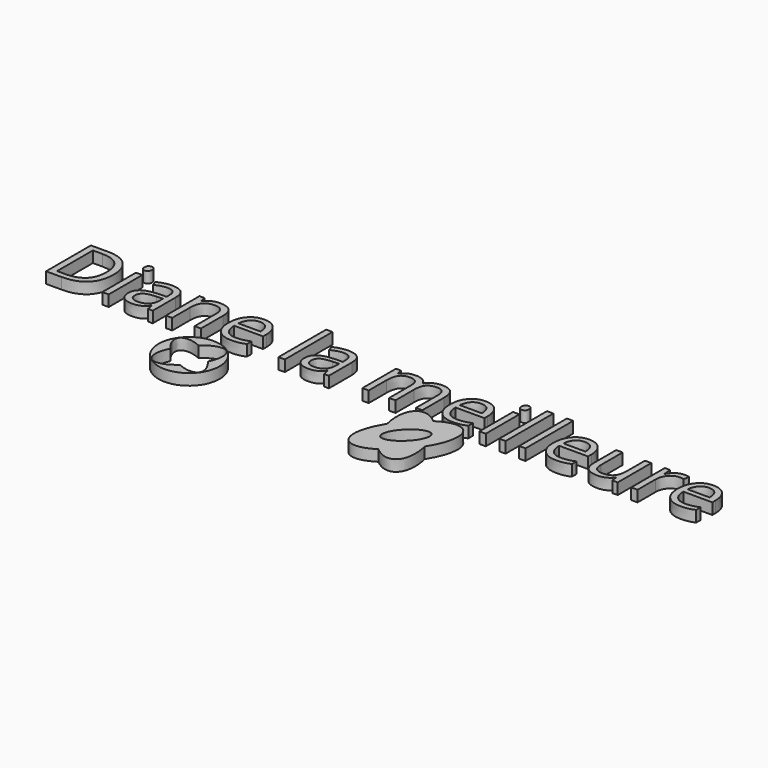
from build123d import *

# Parameters (mm, degrees)
F0_R         = 8.3466025543
F0_TEXT_SIZE = 21.4475266855
F1_DEPTH     = 3.048


# Not quite as in the source:
# - Text() gives the source's letters only with a copy of the font that has no kerning and outlines rounded to 1/6400 em; it was checked with that copy


with BuildPart() as f1:
    # F0 (on Top) → F1 (new body)
    with BuildSketch(Plane.XY):
        with Locations((-38.1957553327, 6.9755995646)):
            Circle(F0_R)
        with BuildLine():
            add(Edge.make_bspline(
                [(-31.5405130386, 2.1061094012), (-30.3175795801, 3.7775202066), (-33.1948879087, 7.1133897692)],
                knots=[0, 0, 0, 1.0706610389, 1.0706610389, 1.0706610389], degree=2, weights=[1, 0.8601000699, 1]))
            add(Edge.make_bspline(
                [(-36.9379521535, 2.2214118859), (-32.788905333, 0.3999034292), (-31.5405130386, 2.1061094012)],
                knots=[5.1943551748, 5.1943551748, 5.1943551748, 6.2831853072, 6.2831853072, 6.2831853072], degree=2, weights=[1, 0.8554303847, 1]))
            add(Edge.make_bspline(
                [(-43.1966227568, 6.83780936), (-51.5075734358, -10.4222102206), (-36.9379521535, 2.2214118859)],
                knots=[1.9673037066, 1.9673037066, 1.9673037066, 4.3401983934, 4.3401983934, 4.3401983934], degree=2, weights=[1, 0.3749556961, 1]))
            add(Edge.make_bspline(
                [(-39.4535585119, 11.7297872433), (-52.2689135199, 17.3559656241), (-43.1966227568, 6.83780936)],
                knots=[2.0527625212, 2.0527625212, 2.0527625212, 4.2122536925, 4.2122536925, 4.2122536925], degree=2, weights=[1, 0.4715527317, 1]))
            add(Edge.make_bspline(
                [(-33.163741231, 13.4682534263), (-35.4280423519, 15.223159111), (-39.4535585119, 11.7297872433)],
                knots=[0, 0, 0, 1.1986057398, 1.1986057398, 1.1986057398], degree=2, weights=[1, 0.8257290436, 1]))
            add(Edge.make_bspline(
                [(-33.1948879087, 7.1133897692), (-30.9580635514, 11.7587827808), (-33.163741231, 13.4682534263)],
                knots=[5.1088963602, 5.1088963602, 5.1088963602, 6.2831853072, 6.2831853072, 6.2831853072], degree=2, weights=[1, 0.8325259928, 1]))
        make_face(mode=Mode.SUBTRACT)
        with BuildLine():
            add(Edge.make_bspline(
                [(21.5702417091, 15.7017175195), (18.5557697987, 18.365754121), (16.3447521627, 17.363846302)],
                knots=[5.4576286446, 5.4576286446, 5.4576286446, 6.2831853072, 6.2831853072, 6.2831853072], degree=2, weights=[1, 0.9160098158, 1]))
            add(Edge.make_bspline(
                [(16.3447521627, 17.363846302), (12.8807705497, 15.7941662569), (14.6476925008, 8.579263006)],
                knots=[0, 0, 0, 1.2026913641, 1.2026913641, 1.2026913641], degree=2, weights=[1, 0.8245750386, 1]))
            add(Edge.make_bspline(
                [(21.5702417091, 15.7017175195), (17.5353416488, 13.1471373461), (14.6476925008, 8.579263006)],
                knots=[0.9615181834, 0.9615181834, 0.9615181834, 1.7930053986, 1.7930053986, 1.7930053986], degree=2, weights=[1, 0.9148162524, 1]))
        make_face()
        with BuildLine():
            add(Edge.make_bspline(
                [(21.5702417091, 15.7017175195), (17.5353416488, 13.1471373461), (14.6476925008, 8.579263006)],
                knots=[0.9615181834, 0.9615181834, 0.9615181834, 1.7930053986, 1.7930053986, 1.7930053986], degree=2, weights=[1, 0.9148162524, 1]))
            add(Edge.make_bspline(
                [(14.6476925008, 8.579263006), (16.2503369357, 2.0351570048), (20.5339913472, -1.7505183903)],
                knots=[1.2026913641, 1.2026913641, 1.2026913641, 2.316035991, 2.316035991, 2.316035991], degree=2, weights=[1, 0.8490180379, 1]))
            add(Edge.make_bspline(
                [(20.5339913472, -1.7505183903), (24.5688914075, 0.8040617832), (27.4565405555, 5.3719361233)],
                knots=[4.103110837, 4.103110837, 4.103110837, 4.9345980522, 4.9345980522, 4.9345980522], degree=2, weights=[1, 0.9148162524, 1]))
            add(Edge.make_bspline(
                [(27.4565405555, 5.3719361233), (25.8538961206, 11.9160421244), (21.5702417091, 15.7017175195)],
                knots=[4.3442840177, 4.3442840177, 4.3442840177, 5.4576286446, 5.4576286446, 5.4576286446], degree=2, weights=[1, 0.8490180379, 1]))
        make_face()
        with BuildLine():
            add(Edge.make_bspline(
                [(17.1563643962, 3.0800073873), (20.3425774952, -0.1063365389), (24.5930991436, 7.3302236901), (28.843620792, 14.7667839192), (21.4068860446, 10.5165676164), (13.9701512972, 6.2663513136), (17.1563643962, 3.0800073873)],
                knots=[0, 0, 0, 2.0943951024, 2.0943951024, 4.1887902048, 4.1887902048, 6.2831853072, 6.2831853072, 6.2831853072], degree=2, weights=[1, 0.5, 1, 0.5, 1, 0.5, 1]))
        make_face(mode=Mode.SUBTRACT)
        with BuildLine():
            add(Edge.make_bspline(
                [(14.6476925008, 8.579263006), (16.2503369357, 2.0351570048), (20.5339913472, -1.7505183903)],
                knots=[1.2026913641, 1.2026913641, 1.2026913641, 2.316035991, 2.316035991, 2.316035991], degree=2, weights=[1, 0.8490180379, 1]))
            add(Edge.make_bspline(
                [(14.6476925008, 8.579263006), (-0.168217137, -14.8575224175), (20.5339913472, -1.7505183903)],
                knots=[1.7930053986, 1.7930053986, 1.7930053986, 4.103110837, 4.103110837, 4.103110837], degree=2, weights=[1, 0.4038703063, 1]))
        make_face()
        with BuildLine():
            add(Edge.make_bspline(
                [(28.8436170667, 16.7145803571), (26.3372112626, 18.719786301), (21.5702417091, 15.7017175195)],
                knots=[0, 0, 0, 0.9615181834, 0.9615181834, 0.9615181834], degree=2, weights=[1, 0.8866441345, 1]))
            add(Edge.make_bspline(
                [(27.4565405555, 5.3719361233), (25.8538961206, 11.9160421244), (21.5702417091, 15.7017175195)],
                knots=[4.3442840177, 4.3442840177, 4.3442840177, 5.4576286446, 5.4576286446, 5.4576286446], degree=2, weights=[1, 0.8490180379, 1]))
            add(Edge.make_bspline(
                [(27.4565405555, 5.3719361233), (32.6844502088, 13.6417892578), (28.8436170667, 16.7145803571)],
                knots=[4.9345980522, 4.9345980522, 4.9345980522, 6.2831853072, 6.2831853072, 6.2831853072], degree=2, weights=[1, 0.7811481666, 1]))
        make_face()
        with BuildLine():
            add(Edge.make_bspline(
                [(20.5339913472, -1.7505183903), (24.5688914075, 0.8040617832), (27.4565405555, 5.3719361233)],
                knots=[4.103110837, 4.103110837, 4.103110837, 4.9345980522, 4.9345980522, 4.9345980522], degree=2, weights=[1, 0.9148162524, 1]))
            add(Edge.make_bspline(
                [(20.5339913472, -1.7505183903), (31.5946769522, -11.525388472), (27.4565405555, 5.3719361233)],
                knots=[2.316035991, 2.316035991, 2.316035991, 4.3442840177, 4.3442840177, 4.3442840177], degree=2, weights=[1, 0.5283638626, 1]))
        make_face()
        with Locations((-88.3101969957, 18.1446088245)):
            Text('Diane la meilleure', F0_TEXT_SIZE, font='Open Sans', text_align=(TextAlign.LEFT, TextAlign.BOTTOM))
    extrude(amount=F1_DEPTH)


solid = f1.part
